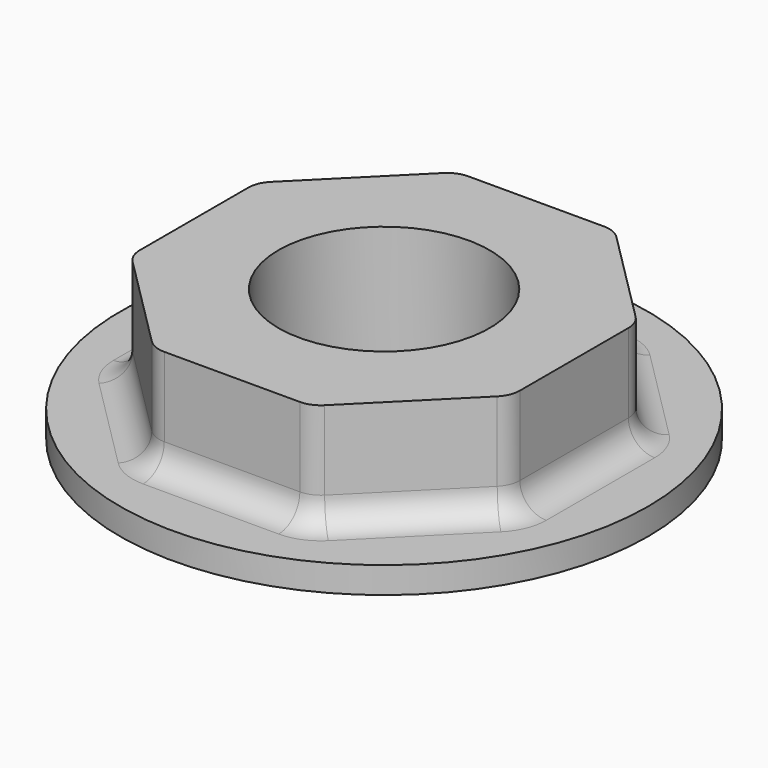
from build123d import *

# Parameters (mm, degrees)
F0_R     = 7.9375
F1_DEPTH = 0.79375
F3_DEPTH = 3.175
F4_R     = 0.79375
F6_D     = 6.35
F6_DEPTH = 19.05
F6_TIP   = 1.9077324654


with BuildPart() as f1:
    # F0 (on Top) → F1 (new body)
    with BuildSketch(Plane.XY):
        Circle(F0_R)
    extrude(amount=F1_DEPTH)

    # F2 (on face) → F3 (join)
    with BuildSketch(Plane.XY.offset(0.79375)):
        Polygon((-5.715, 2.367230509), (-5.715, -2.367230509), (-2.367230509, -5.715), (2.367230509, -5.715), (5.715, -2.367230509), (5.715, 2.367230509), (2.367230509, 5.715), (-2.367230509, 5.715), align=None)
    extrude(amount=F3_DEPTH)

    # F4
    f4_edges = [f1.edges().sort_by_distance(p)[0] for p in [
        (-5.715, -2.367231, 2.38125),
        (-2.367231, -5.715, 2.38125),
        (2.367231, -5.715, 2.38125),
        (5.715, -2.367231, 2.38125),
        (5.715, 2.367231, 2.38125),
        (2.367231, 5.715, 2.38125),
        (-2.367231, 5.715, 2.38125),
        (-5.715, 2.367231, 2.38125),
        (-4.041115, 4.041115, 0.79375),
        (0, 5.715, 0.79375),
        (-5.715, 0, 0.79375),
        (-4.041115, -4.041115, 0.79375),
        (0, -5.715, 0.79375),
        (4.041115, -4.041115, 0.79375),
        (5.715, 0, 0.79375),
        (4.041115, 4.041115, 0.79375),
    ]]
    fillet(f4_edges, radius=F4_R)

    # F6
    with Locations(Plane.XY.offset(3.96875)):
        with Locations((0, 0)):
            Hole(F6_D / 2, depth=F6_DEPTH)
            with Locations((0, 0, -(F6_DEPTH + F6_TIP / 2))):  # 118° drill point
                Cone(0, F6_D / 2, F6_TIP, mode=Mode.SUBTRACT)


solid = f1.part
